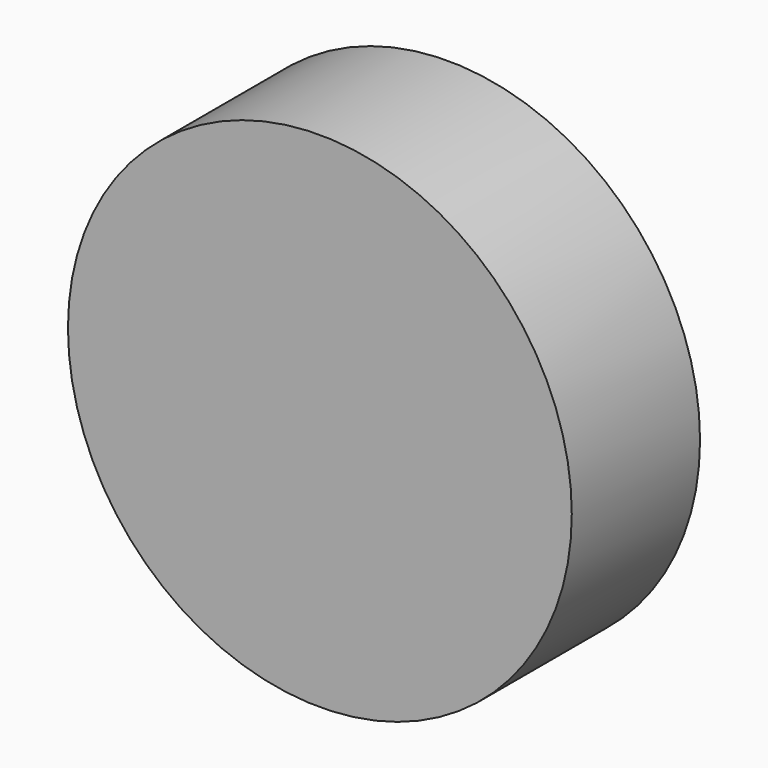
from build123d import *

# Parameters (mm, degrees)
F5_R      = 11
F13_DEPTH = 3.5


# Not quite as in the source:
# - a feature of the source that left no trace in its solid (it failed there, or was rolled back) is left out


with BuildPart() as f13:
    # F5 (on Front) → F13 (new body, symmetric)
    with BuildSketch(Plane.XZ):
        with Locations((0, 12.0977070183)):
            Circle(F5_R)
    extrude(amount=F13_DEPTH, both=True)


solid = f13.part
